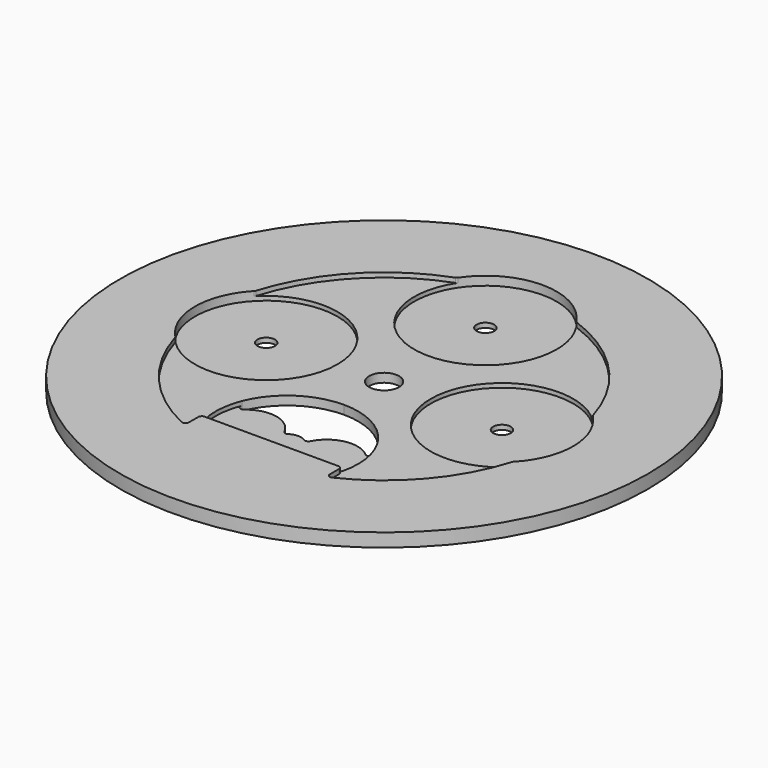
from build123d import *

# Parameters (mm, degrees)
F0_R         = 15
F0_R_2       = 0.5
F0_R_3       = 0.85
F1_DEPTH     = 0.762
F3_DEPTH     = 0.262
F4_R         = 4.05
F5_DEPTH     = 0.5
F6_T4_DEPTH  = 0.6914880487
F6_T9_DEPTH  = 0.6914880487
F6_T11_DEPTH = 0.3832692911
F6_T13_DEPTH = 0.4252513356
F7_R         = 0.3
F8_DEPTH     = 0.3


# Not quite as in the source:
# - a fillet or chamfer that OpenCascade refuses, or shapes differently, is made with other operations: its cross-section is extruded or revolved along the edge and cut away or added


with BuildPart() as f1:
    # F0 (on Top) → F1 (new body)
    with BuildSketch(Plane.XY):
        Circle(F0_R)
        with BuildLine():
            ThreePointArc((-3.7629684096, -5.4024791326), (-2.2734929609, -3.548324336), (0, -2.85))
            ThreePointArc((0, -2.85), (2.2734929609, -3.548324336), (3.7629684096, -5.4024791326))
            ThreePointArc((3.7629684096, -5.4024791326), (3.6929780242, -5.6394712752), (3.4461538031, -5.6275660849))
            ThreePointArc((3.4461538031, -5.6275660849), (1.9616904878, -5.2330123256), (0.7378557396, -6.1612000827))
            ThreePointArc((0.7378557396, -6.1612000827), (0.6097380289, -6.2645935657), (0.4474599736, -6.2368412165))
            ThreePointArc((0.4474599736, -6.2368412165), (0.233958301, -6.1349748283), (0, -6.1))
            ThreePointArc((0, -6.1), (-0.233958301, -6.1349748283), (-0.4474599736, -6.2368412165))
            ThreePointArc((-0.4474599736, -6.2368412165), (-0.6097380289, -6.2645935657), (-0.7378557396, -6.1612000827))
            ThreePointArc((-0.7378557396, -6.1612000827), (-1.9616904878, -5.2330123256), (-3.4461538031, -5.6275660849))
            ThreePointArc((-3.4461538031, -5.6275660849), (-3.6929780242, -5.6394712752), (-3.7629684096, -5.4024791326))
        make_face(mode=Mode.SUBTRACT)
        with Locations((-6.7, 0)):
            Circle(F0_R_2, mode=Mode.SUBTRACT)
        Circle(F0_R_3, mode=Mode.SUBTRACT)
        with Locations((6.7, 0)):
            Circle(F0_R_2, mode=Mode.SUBTRACT)
        with Locations((0, 7.2)):
            Circle(F0_R_2, mode=Mode.SUBTRACT)
    extrude(amount=F1_DEPTH)

    # F2 (on face) → F3 (cut)
    with BuildSketch(Plane.XY.offset(0.762)):
        with BuildLine():
            ThreePointArc((4, -8.8543774485), (4.0930955032, -9.0234082994), (4.2857142857, -9.0350790291))
            ThreePointArc((4.2857142857, -9.0350790291), (0, 10), (-4.2857142857, -9.0350790291))
            ThreePointArc((-4.2857142857, -9.0350790291), (-4.0930955032, -9.0234082994), (-4, -8.8543774485))
            Line((-4, -8.8543774485), (-4, -8.2))
            ThreePointArc((-4, -8.2), (-3.9414213562, -8.0585786438), (-3.8, -8))
            Line((-3.8, -8), (0, -8))
            Line((0, -8), (3.8, -8))
            ThreePointArc((3.8, -8), (3.9414213562, -8.0585786438), (4, -8.2))
            Line((4, -8.2), (4, -8.8543774485))
        make_face()
    extrude(amount=-F3_DEPTH, mode=Mode.SUBTRACT)

    # F4 (on face) → F5 (cut)
    with BuildSketch(Plane.XY.offset(0.762)):
        with Locations((0, 7.2)):
            Circle(F4_R)
        with Locations((6.7, 0)):
            Circle(F4_R)
        with Locations((-6.7, 0)):
            Circle(F4_R)
        with BuildLine():
            ThreePointArc((3.8, -8), (3.8470411203, -8.0056108722), (3.8914428234, -8.02212867))
            ThreePointArc((3.8914428234, -8.02212867), (0, -2.85), (-3.8914428234, -8.02212867))
            ThreePointArc((-3.8914428234, -8.02212867), (-3.8470411203, -8.0056108722), (-3.8, -8))
            Line((-3.8, -8), (3.8, -8))
        make_face()
    extrude(amount=-F5_DEPTH, mode=Mode.SUBTRACT)

    # F6: fillet of radius 0.2 on 8 edges, made by hand


with BuildPart() as f6_tool2:
    # F6_s3 → F6_t4 (new body)
    with BuildSketch(Plane.XY.offset(0.5)):
        with BuildLine():
            ThreePointArc((3.9377859629, -7.8467532468), (3.8671202695, -7.9570838142), (3.7433273968, -8))
            Line((3.7433273968, -8), (3.7433273968, -8.02))
            ThreePointArc((3.7433273968, -8.02), (3.8, -8.02), (3.8822985411, -8.039915803))
            Line((3.8822985411, -8.039915803), (3.910659825, -8.0276700461))
            ThreePointArc((3.910659825, -8.0276700461), (3.9349326547, -7.9398100803), (3.9572318195, -7.8514285714))
            Line((3.9572318195, -7.8514285714), (3.9377859629, -7.8467532468))
        make_face()
    extrude(amount=-F6_T4_DEPTH)

    split(bisect_by=Plane.XY, keep=Keep.TOP)


with BuildPart() as f1_1:
    add(f1.part)

    # F6_t1: union F6_tool2
    add(f6_tool2.part)


with BuildPart() as f6_tool7:
    # F6_s8 → F6_t9 (new body)
    with BuildSketch(Plane.XY.offset(0.5)):
        with BuildLine():
            ThreePointArc((-3.9377859629, -7.8467532468), (-3.8671202695, -7.9570838142), (-3.7433273968, -8))
            Line((-3.7433273968, -8), (-3.7433273968, -8.02))
            ThreePointArc((-3.7433273968, -8.02), (-3.8, -8.02), (-3.8822985411, -8.039915803))
            Line((-3.8822985411, -8.039915803), (-3.910659825, -8.0276700461))
            ThreePointArc((-3.910659825, -8.0276700461), (-3.9349326547, -7.9398100803), (-3.9572318195, -7.8514285714))
            Line((-3.9572318195, -7.8514285714), (-3.9377859629, -7.8467532468))
        make_face()
    extrude(amount=-F6_T9_DEPTH)

    split(bisect_by=Plane.XY, keep=Keep.TOP)


with BuildPart() as f1_2:
    add(f1_1.part)

    # F6_t6: union F6_tool7
    add(f6_tool7.part)

    # F6_s12 → F6_t11 (cut)
    with BuildSketch(Plane.XY.offset(0.5)):
        with BuildLine():
            ThreePointArc((-9.5747366111, 2.8852068953), (-9.5935467273, 2.8420149313), (-9.6219381036, 2.8044211022))
            ThreePointArc((-9.6219381036, 2.8044211022), (-9.6053293925, 2.8216238447), (-9.588619403, 2.8387282266))
            ThreePointArc((-9.588619403, 2.8387282266), (-9.5817061892, 2.8619759788), (-9.5747366111, 2.8852068953))
        make_face()
        with BuildLine():
            ThreePointArc((-9.6219381036, -2.8044211022), (-9.5935467273, -2.8420149313), (-9.5747366111, -2.8852068953))
            ThreePointArc((-9.5747366111, -2.8852068953), (-9.5817061892, -2.8619759788), (-9.588619403, -2.8387282266))
            ThreePointArc((-9.588619403, -2.8387282266), (-9.6053293925, -2.8216238447), (-9.6219381036, -2.8044211022))
        make_face()
        with BuildLine():
            ThreePointArc((9.6219381036, 2.8044211022), (9.5935467273, 2.8420149313), (9.5747366111, 2.8852068953))
            ThreePointArc((9.5747366111, 2.8852068953), (9.5817061892, 2.8619759788), (9.588619403, 2.8387282266))
            ThreePointArc((9.588619403, 2.8387282266), (9.6053293925, 2.8216238447), (9.6219381036, 2.8044211022))
        make_face()
        with BuildLine():
            ThreePointArc((9.6219381036, -2.8044211022), (9.5935467273, -2.8420149313), (9.5747366111, -2.8852068953))
            ThreePointArc((9.5747366111, -2.8852068953), (9.5817061892, -2.8619759788), (9.588619403, -2.8387282266))
            ThreePointArc((9.588619403, -2.8387282266), (9.6053293925, -2.8216238447), (9.6219381036, -2.8044211022))
        make_face()
    extrude(amount=F6_T11_DEPTH, mode=Mode.SUBTRACT)

    # F6_s14 → F6_t13 (cut)
    with BuildSketch(Plane.XY.offset(0.5)):
        with BuildLine():
            ThreePointArc((3.4582244159, 9.3829997277), (3.4038059187, 9.4134107296), (3.3613941322, 9.4590992647))
            ThreePointArc((3.3613941322, 9.4590992647), (3.3792435663, 9.4323111163), (3.3968795208, 9.4053819444))
            ThreePointArc((3.3968795208, 9.4053819444), (3.427570238, 9.3942409094), (3.4582244159, 9.3829997277))
        make_face()
        with BuildLine():
            ThreePointArc((-3.3613941322, 9.4590992647), (-3.4038059187, 9.4134107296), (-3.4582244159, 9.3829997277))
            ThreePointArc((-3.4582244159, 9.3829997277), (-3.427570238, 9.3942409094), (-3.3968795208, 9.4053819444))
            ThreePointArc((-3.3968795208, 9.4053819444), (-3.3792435663, 9.4323111163), (-3.3613941322, 9.4590992647))
        make_face()
    extrude(amount=F6_T13_DEPTH, mode=Mode.SUBTRACT)

    # F7 (on face) → F8 (cut)
    with BuildSketch(Plane(origin=(0, 0, 0), x_dir=(1, 0, 0), z_dir=(0, 0, -1))):
        with Locations((8.42, -7.15)):
            Circle(F7_R)
        with Locations((-8.42, 7.15)):
            Circle(F7_R)
    extrude(amount=-F8_DEPTH, mode=Mode.SUBTRACT)


solid = f1_2.part
